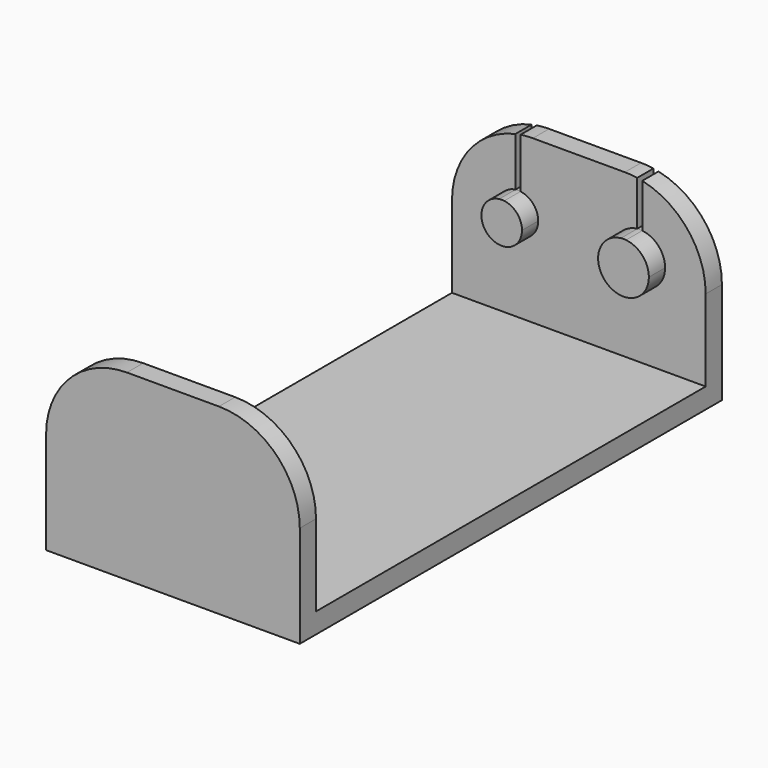
from build123d import *
from build123d import SkipClean  # not in build123d's __all__

# Parameters (mm, degrees)
F0_W     = 25
F0_H     = 52
F1_DEPTH = 18
F2_W     = 25
F2_H     = 48
F3_DEPTH = 16
F4_R     = 7.9669047558
F6_DEPTH = 2
F7_DEPTH = 2


with BuildPart() as f1:
    # F0 (on Top) → F1 (new body)
    with BuildSketch(Plane.XY):
        Rectangle(F0_W, F0_H)
    extrude(amount=F1_DEPTH)

    # F2 (on face) → F3 (cut)
    with BuildSketch(Plane.XY.offset(18)):
        Rectangle(F2_W, F2_H)
    extrude(amount=-F3_DEPTH, mode=Mode.SUBTRACT)

    # F4
    f4_edges = [f1.edges().sort_by_distance(p)[0] for p in [
        (-12.5, 25, 18),
        (12.5, 25, 18),
        (-12.5, -25, 18),
        (12.5, -25, 18),
    ]]
    fillet(f4_edges, radius=F4_R)

    # F5 (on face) → F6 (join)
    with BuildSketch(Plane.XZ.offset(-24)):
        with BuildLine():
            ThreePointArc((-4, 11), (-4.5, 12.3228756555), (-5.75, 12.9843134833))
            ThreePointArc((-5.75, 12.9843134833), (-6, 13), (-6.25, 12.9843134833))
            ThreePointArc((-6.25, 12.9843134833), (-7.3228756555, 9.5), (-4, 11))
        make_face()
        with BuildLine():
            ThreePointArc((5.75, 13.4874685928), (4.3229490169, 9.1459503782), (8.5, 11))
            ThreePointArc((8.5, 11), (7.8540496218, 12.6770509831), (6.25, 13.4874685928))
            ThreePointArc((6.25, 13.4874685928), (6, 13.5), (5.75, 13.4874685928))
        make_face()
    extrude(amount=F6_DEPTH)

    # F5 (on face) → F7 (cut, through all)
    with BuildSketch(Plane.XZ.offset(-24)):
        with BuildLine():
            Line((-5.75, 12.9843134833), (-5.75, 17.9065134474))
            ThreePointArc((-5.75, 17.9065134474), (-6.0007481681, 17.8636486271), (-6.25, 17.8128002159))
            Line((-6.25, 17.8128002159), (-6.25, 12.9843134833))
            ThreePointArc((-6.25, 12.9843134833), (-6, 13), (-5.75, 12.9843134833))
        make_face()
        with BuildLine():
            ThreePointArc((5.75, 13.4874685928), (6, 13.5), (6.25, 13.4874685928))
            Line((6.25, 13.4874685928), (6.25, 17.8128002159))
            ThreePointArc((6.25, 17.8128002159), (6.0007481681, 17.8636486271), (5.75, 17.9065134474))
            Line((5.75, 17.9065134474), (5.75, 13.4874685928))
        make_face()
    with SkipClean():  # cleaning this boolean's faces spoils the solid; the shape is the same uncleaned
        extrude(amount=-F7_DEPTH, mode=Mode.SUBTRACT)


solid = f1.part
